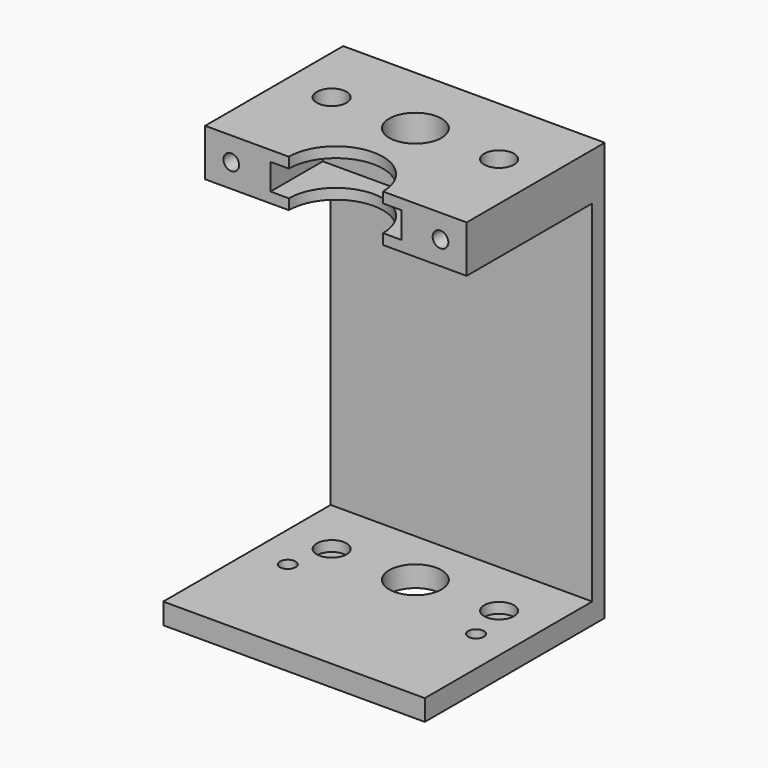
from build123d import *

# Parameters (mm, degrees)
F0_W      = 50
F0_H      = 80
F1_DEPTH  = 3
F2_W      = 50
F2_H      = 4
F3_DEPTH  = 40
F2_H_2    = 9
F4_DEPTH  = 30
F5_W      = 25
F5_H      = 5
F6_DEPTH  = 12.5
F8_DEPTH  = 9
F9_R      = 1.5
F10_DEPTH = 3
F7_R      = 2.85
F11_DEPTH = 78
F7_R_2    = 5
F12_DEPTH = 80
F13_R     = 1.5
F14_DEPTH = 4


with BuildPart() as f1:
    # F0 (on Front) → F1 (new body)
    with BuildSketch(Plane.XZ):
        with Locations((25, 40)):
            Rectangle(F0_W, F0_H)
    extrude(amount=F1_DEPTH)

    # F2 (on face) → F3 (join)
    with BuildSketch(Plane.XZ.offset(3)):
        with Locations((25, 2)):
            Rectangle(F2_W, F2_H)
    extrude(amount=F3_DEPTH)

    # F2 (on face) → F4 (join)
    with BuildSketch(Plane.XZ.offset(3)):
        with Locations((25, 75.5)):
            Rectangle(F2_W, F2_H_2)
    extrude(amount=F4_DEPTH)

    # F5 (on face) → F6 (cut)
    with BuildSketch(Plane.XZ.offset(33)):
        with Locations((25, 75.5)):
            Rectangle(F5_W, F5_H)
    extrude(amount=-F6_DEPTH, mode=Mode.SUBTRACT)

    # F7 (on face) → F8 (cut)
    with BuildSketch(Plane.XY.offset(80)):
        with BuildLine():
            Line((16, -33), (34, -33))
            ThreePointArc((34, -33), (25, -24), (16, -33))
        make_face()
    extrude(amount=-F8_DEPTH, mode=Mode.SUBTRACT)

    # F9 (on face) → F10 (cut)
    with BuildSketch(Plane.XZ.offset(33)):
        with Locations((5, 75.5)):
            Circle(F9_R)
        with Locations((45, 75.5)):
            Circle(F9_R)
    extrude(amount=-F10_DEPTH, mode=Mode.SUBTRACT)

    # F7 (on face) → F11 (cut)
    with BuildSketch(Plane.XY.offset(80)):
        with Locations((9, -14)):
            Circle(F7_R)
        with Locations((41, -14)):
            Circle(F7_R)
    extrude(amount=-F11_DEPTH, mode=Mode.SUBTRACT)

    # F7 (on face) → F12 (cut)
    with BuildSketch(Plane.XY.offset(80)):
        with Locations((25, -14)):
            Circle(F7_R_2)
    extrude(amount=-F12_DEPTH, mode=Mode.SUBTRACT)

    # F13 (on face) → F14 (cut)
    with BuildSketch(Plane.XY.offset(4)):
        with Locations((7, -22)):
            Circle(F13_R)
        with Locations((43, -22)):
            Circle(F13_R)
    extrude(amount=-F14_DEPTH, mode=Mode.SUBTRACT)


solid = f1.part
